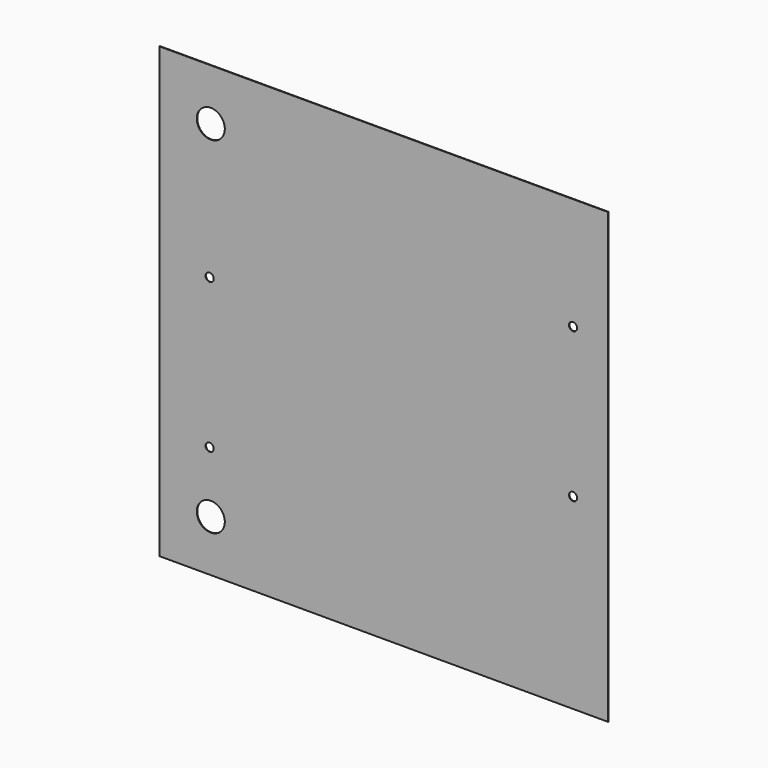
from build123d import *

# Parameters (mm, degrees)
F0_W     = 609.6
F0_H     = 609.6
F1_DEPTH = 0.79375
F2_R     = 5.55625
F3_DEPTH = 25.4
F4_R     = 19.05
F5_DEPTH = 25.4


# Not quite as in the source:
# - a feature names something its author has since deleted; it is built from what else it names


with BuildPart() as f1:
    # F0 (on Front) → F1 (new body)
    with BuildSketch(Plane.XZ):
        with Locations((304.8, 304.8)):
            Rectangle(F0_W, F0_H)
    extrude(amount=F1_DEPTH)

    # F2 (on face) → F3 (cut)
    with BuildSketch(Plane.XZ.offset(0.79375)):
        with Locations((68.2625, 355.6)):
            Circle(F2_R)
        with Locations((68.2625, 152.4)):
            Circle(F2_R)
        with Locations((561.975, 254)):
            Circle(F2_R)
        with Locations((561.975, 457.2)):
            Circle(F2_R)
    extrude(amount=-F3_DEPTH, mode=Mode.SUBTRACT)

    # F4 (on face) → F5 (cut)
    with BuildSketch(Plane.XZ.offset(0.79375)):
        with Locations((69.85, 69.85)):
            Circle(F4_R)
        with Locations((69.85, 539.75)):
            Circle(F4_R)
    extrude(amount=-F5_DEPTH, mode=Mode.SUBTRACT)


solid = f1.part
